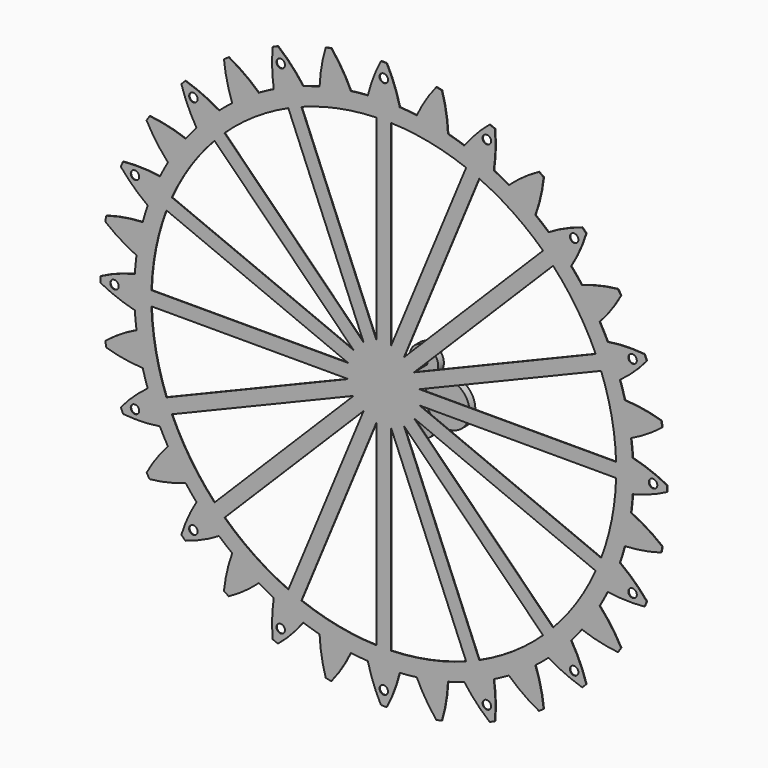
from build123d import *

# Parameters (mm, degrees)
F1_R     = 50.3571046844
F1_R_2   = 13.2254890704
F2_DEPTH = 25
F1_R_3   = 78.4317775594
F1_R_4   = 43.295688096
F1_R_5   = 34.859510012
F1_R_6   = 50.7964382241
F1_R_7   = 35.7797543331
F3_DEPTH = 200
F4_R     = 15
F5_DEPTH = 2
F6_COUNT = 16


with BuildPart() as f2:
    # F1 (on face) → F2 (new body)
    with BuildSketch(Plane.XZ):
        Circle(F1_R)
        Circle(F1_R_2, mode=Mode.SUBTRACT)
    extrude(amount=F2_DEPTH)

    # F1 (on face) → F3 (join)
    with BuildSketch(Plane.XZ):
        Circle(F1_R_2)
    extrude(amount=F3_DEPTH)


with BuildPart() as f2b:
    # F1 (on face) → F2, piece 2 (new body)
    with BuildSketch(Plane.XZ):
        with Locations((83.0070003867, -106.5655499697)):
            Circle(F1_R_3)
    extrude(amount=F2_DEPTH)


with BuildPart() as f2c:
    # F1 (on face) → F2, piece 3 (new body)
    with BuildSketch(Plane.XZ):
        with Locations((-6.8326536566, -197.5570172071)):
            Circle(F1_R_4)
    extrude(amount=F2_DEPTH)


with BuildPart() as f2d:
    # F1 (on face) → F2, piece 4 (new body)
    with BuildSketch(Plane.XZ):
        with Locations((-87.4579995871, -172.2176074982)):
            Circle(F1_R_5)
    extrude(amount=F2_DEPTH)


with BuildPart() as f2e:
    # F1 (on face) → F2, piece 5 (new body)
    with BuildSketch(Plane.XZ):
        with Locations((-174.9940812588, -136.5121006966)):
            Circle(F1_R_6)
    extrude(amount=F2_DEPTH)


with BuildPart() as f2f:
    # F1 (on face) → F2, piece 6 (new body)
    with BuildSketch(Plane.XZ):
        with Locations((-174.9940812588, -40.9134700894)):
            Circle(F1_R_7)
    extrude(amount=F2_DEPTH)


with BuildPart() as f5:
    # F4 (on face) → F5 (new body)
    with BuildSketch(Plane.XZ.offset(200)):
        with BuildLine():
            ThreePointArc((13.2254890704, 0), (13.1618047257, 1.2963246181), (12.9713650064, 2.5801649216))
            Line((12.9713650064, 2.5801649216), (0, 0))
            Line((0, 0), (12.9713650064, -2.5801649216))
            ThreePointArc((12.9713650064, -2.5801649216), (13.1618047257, -1.2963246181), (13.2254890704, 0))
        make_face()
        with BuildLine():
            ThreePointArc((999.9499987499, -10), (999.9874996094, -5.0000625027), (1000, 0))
            ThreePointArc((1000, 0), (999.9874996094, 5.0000625027), (999.9499987499, 10))
            ThreePointArc((999.9499987499, 10), (940.4986437371, 36.8746811277), (878.2000714994, 56.25508349))
            ThreePointArc((878.2000714994, 56.25508349), (877.1095870589, 71.2655056068), (875.7625594715, 86.25508349))
            ThreePointArc((875.7625594715, 86.25508349), (874.1593827254, 101.2194328831), (872.3005257288, 116.1541769085))
            ThreePointArc((872.3005257288, 116.1541769085), (929.621119432, 147.3160387928), (982.6871431333, 185.2727144521))
            ThreePointArc((982.6871431333, 185.2727144521), (981.7484840078, 190.1838956071), (980.7852804032, 195.0903220161))
            Line((980.7852804032, 195.0903220161), (804.2439299306, 159.9740640532))
            ThreePointArc((804.2439299306, 159.9740640532), (814.731276031, 92.8059688646), (819.6188138397, 25))
            Line((819.6188138397, 25), (125.6834873031, 25))
            Line((125.6834873031, 25), (12.9713650064, 2.5801649216))
            ThreePointArc((12.9713650064, 2.5801649216), (13.1618047257, 1.2963246181), (13.2254890704, 0))
            ThreePointArc((13.2254890704, 0), (13.1618047257, -1.2963246181), (12.9713650064, -2.5801649216))
            Line((12.9713650064, -2.5801649216), (125.6834873031, -25))
            Line((125.6834873031, -25), (819.6188138397, -25))
            ThreePointArc((819.6188138397, -25), (814.731276031, -92.8059688646), (804.2439299306, -159.9740640532))
            Line((804.2439299306, -159.9740640532), (980.7852804032, -195.0903220161))
            ThreePointArc((980.7852804032, -195.0903220161), (981.7484840078, -190.1838956071), (982.6871431333, -185.2727144521))
            ThreePointArc((982.6871431333, -185.2727144521), (929.621119432, -147.3160387928), (872.3005257288, -116.1541769085))
            ThreePointArc((872.3005257288, -116.1541769085), (874.1593827254, -101.2194328831), (875.7625594715, -86.25508349))
            ThreePointArc((875.7625594715, -86.25508349), (877.1095870589, -71.2655056068), (878.2000714994, -56.25508349))
            ThreePointArc((878.2000714994, -56.25508349), (940.4986437371, -36.8746811277), (999.9499987499, -10))
        make_face()
        with Locations((950, 0)):
            Circle(F4_R, mode=Mode.SUBTRACT)
    extrude(amount=F5_DEPTH)

    # F6: F5 ×16 about axis
    f6_axis = Axis((0, 0, 0), (0, -1, 0))


with BuildPart() as f5_1:
    add(f5.part)
    for i in range(1, F6_COUNT):
        add(f5.part.rotate(f6_axis, i * 360 / F6_COUNT))


solid = Compound([f2.part, f2b.part, f2c.part, f2d.part, f2e.part, f2f.part, f5_1.part])
